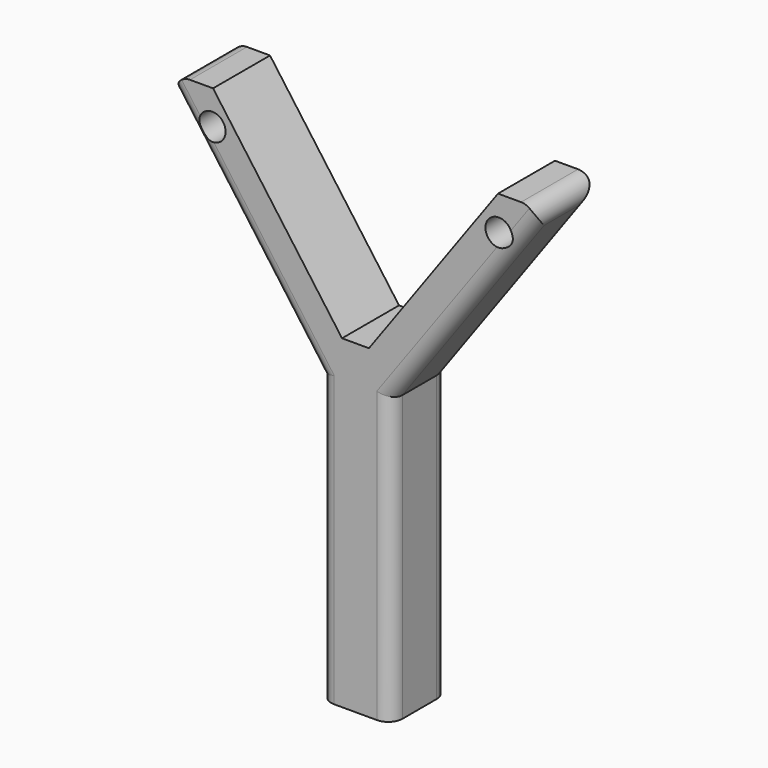
from build123d import *

# Parameters (mm, degrees)
F1_DEPTH     = 25.4
F3_DEPTH     = 25.401
F4_T1_DEPTH  = 75.1590131963
F4_T6_DEPTH  = 127
F4_T11_DEPTH = 127
F4_T16_DEPTH = 127
F4_T21_DEPTH = 127
F4_T26_DEPTH = 121.344223221
F4_T31_DEPTH = 121.344223221
F4_T36_DEPTH = 121.344223221
F4_T41_DEPTH = 121.344223221
F4_T47_DEPTH = 121.344223221
F4_T51_DEPTH = 127
F4_T58_DEPTH = 127
F4_T62_DEPTH = 121.344223221
F4_T69_DEPTH = 121.344223221
F4_T73_DEPTH = 127
F4_T80_DEPTH = 127
F4_T84_DEPTH = 121.344223221


# Not quite as in the source:
# - a fillet or chamfer that OpenCascade refuses, or shapes differently, is made with other operations: its cross-section is extruded or revolved along the edge and cut away or added


with BuildPart() as f1:
    # F0 (on Front) → F1 (new body)
    with BuildSketch(Plane.XZ):
        Polygon((4.8083475167, 0), (0, 0), (-4.8083475167, 0), (-50.8, 63.5), (-68.9793676138, 63.5), (-12.7, -14.2040973853), (-12.7, -115.8040973853), (0, -115.8040973853), (12.7, -115.8040973853), (12.7, -14.2040973853), (68.9793676138, 63.5), (50.8, 63.5), align=None)
    extrude(amount=F1_DEPTH)

    # F2 (on face) → F3 (cut, through all)
    with BuildSketch(Plane(origin=(0, 0, 0), x_dir=(-1, 0, 0), z_dir=(0, 1, 0))):
        with BuildLine():
            ThreePointArc((-46.3238090676, 51.3453096211), (-51.0863090676, 56.1078096211), (-55.8488090676, 51.3453096211))
            Line((-55.8488090676, 51.3453096211), (-46.3238090676, 51.3453096211))
        make_face()
        with BuildLine():
            Line((-46.3238090676, 51.3453096211), (-55.8488090676, 51.3453096211))
            ThreePointArc((-55.8488090676, 51.3453096211), (-51.0863090676, 46.5828096211), (-46.3238090676, 51.3453096211))
        make_face()
        with BuildLine():
            ThreePointArc((55.8488090676, 51.3453096211), (51.0863090676, 56.1078096211), (46.3238090676, 51.3453096211))
            Line((46.3238090676, 51.3453096211), (55.8488090676, 51.3453096211))
        make_face()
        with BuildLine():
            Line((55.8488090676, 51.3453096211), (46.3238090676, 51.3453096211))
            ThreePointArc((46.3238090676, 51.3453096211), (51.0863090676, 46.5828096211), (55.8488090676, 51.3453096211))
        make_face()
    extrude(amount=-F3_DEPTH, mode=Mode.SUBTRACT)

    # F4: fillet of radius 5.08 on 10 edges, made by hand

    # F4_s2 → F4_t1 (cut)
    with BuildSketch(Plane.XZ.offset(-24.8795065982)):
        with BuildLine():
            ThreePointArc((-63.1417971968, 55.440152148), (-63.552165901, 60.7296290732), (-59.0275649745, 63.5))
            Line((-59.0275649745, 63.5), (-68.9793676138, 63.5))
            Line((-68.9793676138, 63.5), (-63.1417971968, 55.440152148))
        make_face()
        with BuildLine():
            ThreePointArc((63.1417971968, 55.440152148), (63.552165901, 60.7296290732), (59.0275649745, 63.5))
            Line((59.0275649745, 63.5), (68.9793676138, 63.5))
            Line((68.9793676138, 63.5), (63.1417971968, 55.440152148))
        make_face()
    extrude(amount=F4_T1_DEPTH, mode=Mode.SUBTRACT)


with BuildPart() as f4_tool4:
    # F4_s5 → F4_t6 (new body)
    with BuildSketch(Plane.XY.offset(-128.5040973853)):
        with BuildLine():
            ThreePointArc((12.7, -5.08), (11.2121024484, -1.4878975516), (7.62, 0))
            Line((7.62, 0), (12.7, 0))
            Line((12.7, 0), (12.7, -5.08))
        make_face()
    extrude(amount=F4_T6_DEPTH)

    split(bisect_by=Plane(origin=(15.0780779602, 0, -10.9207200262), x_dir=(0, 1, 0), z_dir=(0.8098882327, 0, -0.5865842228)), keep=Keep.TOP)


with BuildPart() as f1_1:
    add(f1.part)

    # F4_t3: cut F4_tool4
    add(f4_tool4.part, mode=Mode.SUBTRACT)


with BuildPart() as f4_tool9:
    # F4_s10 → F4_t11 (new body)
    with BuildSketch(Plane.XY.offset(-1.5040973853)):
        with BuildLine():
            ThreePointArc((-7.62, 0), (-11.2121024484, -1.4878975516), (-12.7, -5.08))
            Line((-12.7, -5.08), (-12.7, 0))
            Line((-12.7, 0), (-7.62, 0))
        make_face()
    extrude(amount=-F4_T11_DEPTH)

    split(bisect_by=Plane(origin=(-15.0780779602, 0, -10.9207200262), x_dir=(0, 1, 0), z_dir=(-0.8098882327, 0, -0.5865842228)), keep=Keep.TOP)


with BuildPart() as f1_2:
    add(f1_1.part)

    # F4_t8: cut F4_tool9
    add(f4_tool9.part, mode=Mode.SUBTRACT)


with BuildPart() as f4_tool14:
    # F4_s15 → F4_t16 (new body)
    with BuildSketch(Plane.XY.offset(-128.5040973853)):
        with BuildLine():
            ThreePointArc((12.7, -20.32), (11.2121024484, -23.9121024484), (7.62, -25.4))
            Line((7.62, -25.4), (12.7, -25.4))
            Line((12.7, -25.4), (12.7, -20.32))
        make_face()
    extrude(amount=F4_T16_DEPTH)

    split(bisect_by=Plane(origin=(15.0780779602, 0, -10.9207200262), x_dir=(0, 1, 0), z_dir=(0.8098882327, 0, -0.5865842228)), keep=Keep.TOP)


with BuildPart() as f1_3:
    add(f1_2.part)

    # F4_t13: cut F4_tool14
    add(f4_tool14.part, mode=Mode.SUBTRACT)


with BuildPart() as f4_tool19:
    # F4_s20 → F4_t21 (new body)
    with BuildSketch(Plane.XY.offset(-1.5040973853)):
        with BuildLine():
            ThreePointArc((-7.62, -25.4), (-11.2121024484, -23.9121024484), (-12.7, -20.32))
            Line((-12.7, -20.32), (-12.7, -25.4))
            Line((-12.7, -25.4), (-7.62, -25.4))
        make_face()
    extrude(amount=-F4_T21_DEPTH)

    split(bisect_by=Plane(origin=(-15.0780779602, 0, -10.9207200262), x_dir=(0, 1, 0), z_dir=(-0.8098882327, 0, -0.5865842228)), keep=Keep.TOP)


with BuildPart() as f1_4:
    add(f1_3.part)

    # F4_t18: cut F4_tool19
    add(f4_tool19.part, mode=Mode.SUBTRACT)


with BuildPart() as f4_tool24:
    # F4_s25 → F4_t26 (new body)
    with BuildSketch(Plane(origin=(-9.8276975902, 0, -13.5689579148), x_dir=(0, 1, 0), z_dir=(0.5865842228, 0, 0.8098882327))):
        with BuildLine():
            ThreePointArc((-20.32, -18.6174799816), (-23.9121024484, -17.12958243), (-25.4, -13.5374799816))
            Line((-25.4, -13.5374799816), (-25.4, -18.6174799816))
            Line((-25.4, -18.6174799816), (-20.32, -18.6174799816))
        make_face()
    extrude(amount=F4_T26_DEPTH)

    split(bisect_by=Plane.YZ.offset(12.7), keep=Keep.TOP)


with BuildPart() as f1_5:
    add(f1_4.part)

    # F4_t23: cut F4_tool24
    add(f4_tool24.part, mode=Mode.SUBTRACT)


with BuildPart() as f4_tool29:
    # F4_s30 → F4_t31 (new body)
    with BuildSketch(Plane(origin=(-9.8276975902, 0, -13.5689579148), x_dir=(0, 1, 0), z_dir=(0.5865842228, 0, 0.8098882327))):
        with BuildLine():
            ThreePointArc((-5.08, -18.6174799816), (-1.4878975516, -17.12958243), (0, -13.5374799816))
            Line((0, -13.5374799816), (0, -18.6174799816))
            Line((0, -18.6174799816), (-5.08, -18.6174799816))
        make_face()
    extrude(amount=F4_T31_DEPTH)

    split(bisect_by=Plane.YZ.offset(12.7), keep=Keep.TOP)


with BuildPart() as f1_6:
    add(f1_5.part)

    # F4_t28: cut F4_tool29
    add(f4_tool29.part, mode=Mode.SUBTRACT)


with BuildPart() as f4_tool34:
    # F4_s35 → F4_t36 (new body)
    with BuildSketch(Plane(origin=(-61.3509092836, 0, 84.7063005819), x_dir=(0, 1, 0), z_dir=(0.5865842228, 0, -0.8098882327))):
        with BuildLine():
            ThreePointArc((-25.4, -13.5374799816), (-23.9121024484, -17.12958243), (-20.32, -18.6174799816))
            Line((-20.32, -18.6174799816), (-25.4, -18.6174799816))
            Line((-25.4, -18.6174799816), (-25.4, -13.5374799816))
        make_face()
    extrude(amount=F4_T36_DEPTH)

    split(bisect_by=Plane.YZ.offset(-12.7), keep=Keep.BOTTOM)


with BuildPart() as f1_7:
    add(f1_6.part)

    # F4_t33: cut F4_tool34
    add(f4_tool34.part, mode=Mode.SUBTRACT)


with BuildPart() as f4_tool39:
    # F4_s40 → F4_t41 (new body)
    with BuildSketch(Plane(origin=(-61.3509092836, 0, 84.7063005819), x_dir=(0, 1, 0), z_dir=(0.5865842228, 0, -0.8098882327))):
        with BuildLine():
            ThreePointArc((0, -13.5374799816), (-1.4878975516, -17.12958243), (-5.08, -18.6174799816))
            Line((-5.08, -18.6174799816), (0, -18.6174799816))
            Line((0, -18.6174799816), (0, -13.5374799816))
        make_face()
    extrude(amount=F4_T41_DEPTH)

    split(bisect_by=Plane.YZ.offset(-12.7), keep=Keep.BOTTOM)


with BuildPart() as f1_8:
    add(f1_7.part)

    # F4_t38: cut F4_tool39
    add(f4_tool39.part, mode=Mode.SUBTRACT)


with BuildPart() as f4_tool45:
    # F4_s46 → F4_t47 (new body)
    with BuildSketch(Plane(origin=(-9.8276975902, 0, -13.5689579148), x_dir=(0, 1, 0), z_dir=(0.5865842228, 0, 0.8098882327))):
        with BuildLine():
            ThreePointArc((-5.08, -18.6174799816), (-1.4878975516, -17.12958243), (0, -13.5374799816))
            Line((0, -13.5374799816), (0, -18.6174799816))
            Line((0, -18.6174799816), (-5.08, -18.6174799816))
        make_face()
    extrude(amount=F4_T47_DEPTH)

    split(bisect_by=Plane.YZ.offset(12.7), keep=Keep.BOTTOM)


with BuildPart() as f4_tool49:
    # F4_s50 → F4_t51 (new body)
    with BuildSketch(Plane.XY.offset(-128.5040973853)):
        with BuildLine():
            ThreePointArc((12.7, -5.08), (11.2121024484, -1.4878975516), (7.62, 0))
            Line((7.62, 0), (12.7, 0))
            Line((12.7, 0), (12.7, -5.08))
        make_face()
    extrude(amount=F4_T51_DEPTH)

    split(bisect_by=Plane(origin=(15.0780779602, 0, -10.9207200262), x_dir=(0, 1, 0), z_dir=(-0.8098882327, 0, 0.5865842228)), keep=Keep.TOP)


with BuildPart() as f4_tool45_1:
    add(f4_tool45.part)

    # F4_t53: intersect F4_tool49
    add(f4_tool49.part, mode=Mode.INTERSECT)


with BuildPart() as f1_9:
    add(f1_8.part)

    # F4_t43: cut F4_tool45
    add(f4_tool45_1.part, mode=Mode.SUBTRACT)


with BuildPart() as f4_tool56:
    # F4_s57 → F4_t58 (new body)
    with BuildSketch(Plane.XY.offset(-1.5040973853)):
        with BuildLine():
            ThreePointArc((-7.62, 0), (-11.2121024484, -1.4878975516), (-12.7, -5.08))
            Line((-12.7, -5.08), (-12.7, 0))
            Line((-12.7, 0), (-7.62, 0))
        make_face()
    extrude(amount=-F4_T58_DEPTH)

    split(bisect_by=Plane(origin=(-15.0780779602, 0, -10.9207200262), x_dir=(0, 1, 0), z_dir=(0.8098882327, 0, 0.5865842228)), keep=Keep.TOP)


with BuildPart() as f4_tool60:
    # F4_s61 → F4_t62 (new body)
    with BuildSketch(Plane(origin=(-61.3509092836, 0, 84.7063005819), x_dir=(0, 1, 0), z_dir=(0.5865842228, 0, -0.8098882327))):
        with BuildLine():
            ThreePointArc((0, -13.5374799816), (-1.4878975516, -17.12958243), (-5.08, -18.6174799816))
            Line((-5.08, -18.6174799816), (0, -18.6174799816))
            Line((0, -18.6174799816), (0, -13.5374799816))
        make_face()
    extrude(amount=F4_T62_DEPTH)

    split(bisect_by=Plane.YZ.offset(-12.7), keep=Keep.TOP)


with BuildPart() as f4_tool56_1:
    add(f4_tool56.part)

    # F4_t64: intersect F4_tool60
    add(f4_tool60.part, mode=Mode.INTERSECT)


with BuildPart() as f1_10:
    add(f1_9.part)

    # F4_t54: cut F4_tool56
    add(f4_tool56_1.part, mode=Mode.SUBTRACT)


with BuildPart() as f4_tool67:
    # F4_s68 → F4_t69 (new body)
    with BuildSketch(Plane(origin=(-9.8276975902, 0, -13.5689579148), x_dir=(0, 1, 0), z_dir=(0.5865842228, 0, 0.8098882327))):
        with BuildLine():
            ThreePointArc((-20.32, -18.6174799816), (-23.9121024484, -17.12958243), (-25.4, -13.5374799816))
            Line((-25.4, -13.5374799816), (-25.4, -18.6174799816))
            Line((-25.4, -18.6174799816), (-20.32, -18.6174799816))
        make_face()
    extrude(amount=F4_T69_DEPTH)

    split(bisect_by=Plane.YZ.offset(12.7), keep=Keep.BOTTOM)


with BuildPart() as f4_tool71:
    # F4_s72 → F4_t73 (new body)
    with BuildSketch(Plane.XY.offset(-128.5040973853)):
        with BuildLine():
            ThreePointArc((12.7, -20.32), (11.2121024484, -23.9121024484), (7.62, -25.4))
            Line((7.62, -25.4), (12.7, -25.4))
            Line((12.7, -25.4), (12.7, -20.32))
        make_face()
    extrude(amount=F4_T73_DEPTH)

    split(bisect_by=Plane(origin=(15.0780779602, 0, -10.9207200262), x_dir=(0, 1, 0), z_dir=(-0.8098882327, 0, 0.5865842228)), keep=Keep.TOP)


with BuildPart() as f4_tool67_1:
    add(f4_tool67.part)

    # F4_t75: intersect F4_tool71
    add(f4_tool71.part, mode=Mode.INTERSECT)


with BuildPart() as f1_11:
    add(f1_10.part)

    # F4_t65: cut F4_tool67
    add(f4_tool67_1.part, mode=Mode.SUBTRACT)


with BuildPart() as f4_tool78:
    # F4_s79 → F4_t80 (new body)
    with BuildSketch(Plane.XY.offset(-1.5040973853)):
        with BuildLine():
            ThreePointArc((-7.62, -25.4), (-11.2121024484, -23.9121024484), (-12.7, -20.32))
            Line((-12.7, -20.32), (-12.7, -25.4))
            Line((-12.7, -25.4), (-7.62, -25.4))
        make_face()
    extrude(amount=-F4_T80_DEPTH)

    split(bisect_by=Plane(origin=(-15.0780779602, 0, -10.9207200262), x_dir=(0, 1, 0), z_dir=(0.8098882327, 0, 0.5865842228)), keep=Keep.TOP)


with BuildPart() as f4_tool82:
    # F4_s83 → F4_t84 (new body)
    with BuildSketch(Plane(origin=(-61.3509092836, 0, 84.7063005819), x_dir=(0, 1, 0), z_dir=(0.5865842228, 0, -0.8098882327))):
        with BuildLine():
            ThreePointArc((-25.4, -13.5374799816), (-23.9121024484, -17.12958243), (-20.32, -18.6174799816))
            Line((-20.32, -18.6174799816), (-25.4, -18.6174799816))
            Line((-25.4, -18.6174799816), (-25.4, -13.5374799816))
        make_face()
    extrude(amount=F4_T84_DEPTH)

    split(bisect_by=Plane.YZ.offset(-12.7), keep=Keep.TOP)


with BuildPart() as f4_tool78_1:
    add(f4_tool78.part)

    # F4_t86: intersect F4_tool82
    add(f4_tool82.part, mode=Mode.INTERSECT)


with BuildPart() as f1_12:
    add(f1_11.part)

    # F4_t76: cut F4_tool78
    add(f4_tool78_1.part, mode=Mode.SUBTRACT)


solid = f1_12.part
